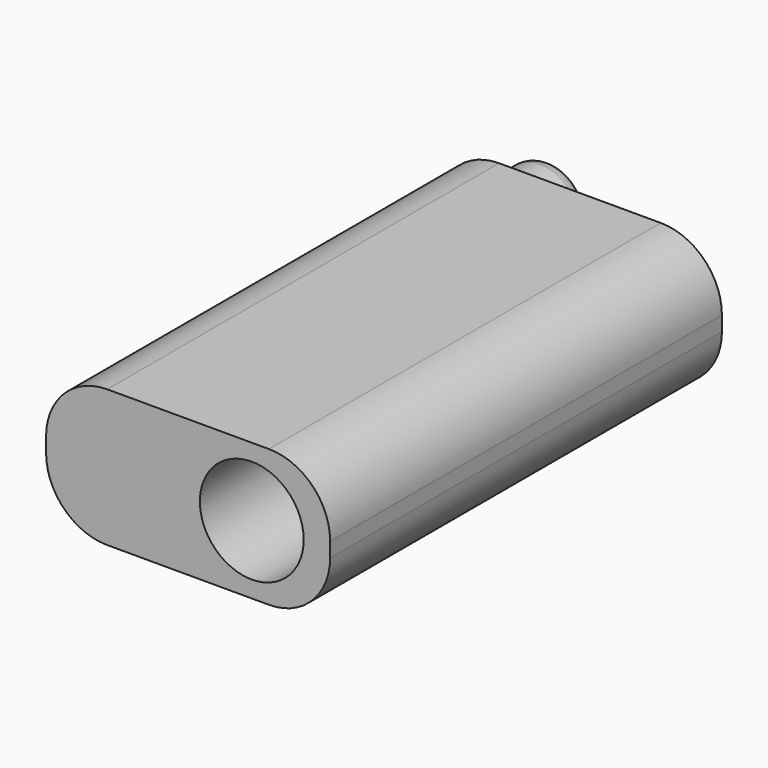
from build123d import *

# Parameters (mm, degrees)
F0_W     = 14.732
F0_H     = 7.112
F0_R     = 2.0066
F0_R_2   = 2.6924
F1_DEPTH = 25.4
F2_DEPTH = 25.401
F3_DEPTH = 4.064
F4_R     = 1.3208
F5_DEPTH = 25.401
F6_R     = 0.762
F7_R     = 3.175


# Not quite as in the source:
# - a feature names something its author has since deleted; it is built from what else it names


with BuildPart() as f1:
    # F0 (on Front) → F1 (new body)
    with BuildSketch(Plane.XZ):
        Rectangle(F0_W, F0_H)
        with Locations((-4.699, 0)):
            Circle(F0_R, mode=Mode.SUBTRACT)
        with Locations((3.302, 0)):
            Circle(F0_R_2, mode=Mode.SUBTRACT)
        with Locations((3.302, 0)):
            Circle(F0_R_2)
        with Locations((-4.699, 0)):
            Circle(F0_R)
    extrude(amount=F1_DEPTH)

    # F0 (on Front) → F2 (cut, through all)
    with BuildSketch(Plane.XZ):
        with Locations((3.302, 0)):
            Circle(F0_R_2)
    extrude(amount=F2_DEPTH, mode=Mode.SUBTRACT)

    # F0 (on Front) → F3 (join)
    with BuildSketch(Plane.XZ):
        with Locations((-4.699, 0)):
            Circle(F0_R)
    extrude(amount=-F3_DEPTH)

    # F4 (on face) → F5 (cut, through all)
    with BuildSketch(Plane.XZ):
        with Locations((3.302, 0)):
            Circle(F4_R)
    extrude(amount=F5_DEPTH, mode=Mode.SUBTRACT)

    # F6
    f6_edges = [f1.edges().sort_by_distance(p)[0] for p in [
        (-6.7056, 4.064, 0),
    ]]
    fillet(f6_edges, radius=F6_R)

    # F7
    f7_edges = [f1.edges().sort_by_distance(p)[0] for p in [
        (7.366, -12.7, 3.556),
        (7.366, -12.7, -3.556),
        (-7.366, -12.7, -3.556),
        (-7.366, -12.7, 3.556),
    ]]
    fillet(f7_edges, radius=F7_R)


solid = f1.part
